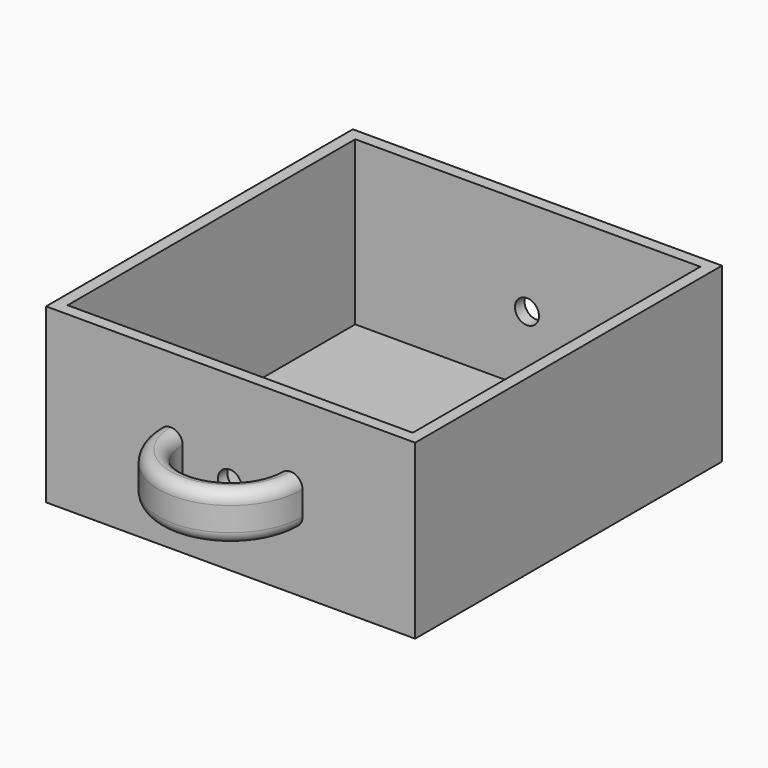
from build123d import *

# Parameters (mm, degrees)
F0_W      = 97.79
F0_H      = 45.72
F1_DEPTH  = 101.6
F2_W      = 91.44
F2_H      = 95.25
F3_DEPTH  = 43.18
F4_W      = 19.05
F4_H      = 6.35
F5_ANGLE  = 180
F7_DEPTH  = 25.4
F8_R      = 3.17499
F10_D     = 6.35
F10_DEPTH = 101.601


# Not quite as in the source:
# - a fillet or chamfer is up to 0.001 mm smaller than in the source, because OpenCascade refuses the exact size


with BuildPart() as f1:
    # F0 (on Front) → F1 (new body)
    with BuildSketch(Plane.XZ):
        with Locations((15.4838143581, 4.6649015626)):
            Rectangle(F0_W, F0_H)
    extrude(amount=-F1_DEPTH)

    # F2 (on face) → F3 (cut)
    with BuildSketch(Plane.XY.offset(27.5249015626)):
        with Locations((15.4838143581, 50.8)):
            Rectangle(F2_W, F2_H)
    extrude(amount=-F3_DEPTH, mode=Mode.SUBTRACT)

    # F4 (on face) → F5 (revolve)
    with BuildSketch(Plane.XZ):
        with Locations((5.9588143581, 6.8874015626)):
            Rectangle(F4_W, F4_H)
        with Locations((5.9588143581, 0.5374015626)):
            Rectangle(F4_W, F4_H)
    revolve(axis=Axis((15.4838143581, 0, 3.7124015626), (0, 0, 1)), revolution_arc=F5_ANGLE)

    # F6 (on face) → F7 (cut)
    with BuildSketch(Plane.XY.offset(10.0624015626)):
        with BuildLine():
            Line((28.1838143581, 0), (2.7838143581, 0))
            ThreePointArc((2.7838143581, 0), (15.4838143581, -12.7), (28.1838143581, 0))
        make_face()
    extrude(amount=-F7_DEPTH, mode=Mode.SUBTRACT)

    # F8 (radius 3.175 in the source; OpenCascade refuses exactly that, so slightly less here)
    f8_edges = [f1.edges().sort_by_distance(p)[0] for p in [
        (15.483814, -19.05, 10.062402),
        (15.483814, -12.7, 10.062402),
        (15.483814, -19.05, -2.637598),
        (15.483814, -12.7, -2.637598),
    ]]
    fillet(f8_edges, radius=F8_R)

    # F10 (through all, one way)
    with BuildSketch(Plane.XZ):
        with Locations((15.265179798, 2.1249015626)):
            Circle(F10_D / 2)
    extrude(amount=-F10_DEPTH, mode=Mode.SUBTRACT)


solid = f1.part
